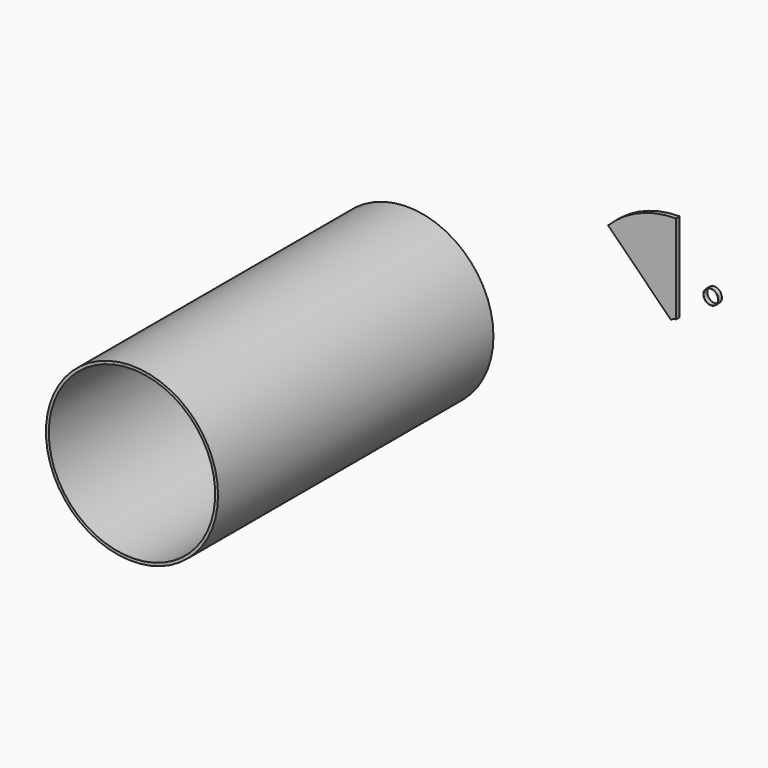
from build123d import *

# Parameters (mm, degrees)
F0_R     = 19.05
F1_DEPTH = 76.2
F3_D     = 36.83
F3_DEPTH = 76.2
F3_TIP   = 11.0648482994
F5_DEPTH = 1.016
F8_R     = 1.651
F8_R_2   = 1.5875
F9_DEPTH = 1.016


# Not quite as in the source:
# - a feature of the source that left no trace in its solid (it failed there, or was rolled back) is left out
# - a length typed as a fraction of an inch, garbled in the dataset ("3 / 203.2 mm" for 3/8 in), is restored
# - a feature names something its author has since deleted; it is built from what else it names


with BuildPart() as f1:
    # F0 (on Front) → F1 (new body)
    with BuildSketch(Plane.XZ):
        with Locations((-13.1577122957, 38.5967120528)):
            Circle(F0_R)
    extrude(amount=F1_DEPTH)

    # F3
    with Locations(Plane.XZ.offset(76.2)):
        with Locations((-13.1577122957, 38.5967120528)):
            Hole(F3_D / 2, depth=F3_DEPTH)
            with Locations((0, 0, -(F3_DEPTH + F3_TIP / 2))):  # 118° drill point
                Cone(0, F3_D / 2, F3_TIP, mode=Mode.SUBTRACT)


with BuildPart() as f5:
    # F4 (on Front) → F5 (new body)
    with BuildSketch(Plane.XZ):
        with BuildLine():
            Line((47.1229890541, 55.69569515), (47.1229890541, 75.38069515))
            ThreePointArc((47.1229890541, 75.38069515), (38.9823557391, 73.7614225053), (32.0810600513, 69.1501241528))
            Line((32.0810600513, 69.1501241528), (46.0004570389, 55.2307271651))
            ThreePointArc((46.0004570389, 55.2307271651), (46.5154791052, 55.5748539078), (47.1229890541, 55.69569515))
        make_face()
    extrude(amount=F5_DEPTH)


with BuildPart() as f9:
    # F8 (on Front) → F9 (new body)
    with BuildSketch(Plane.XZ):
        with Locations((54.8101738095, 62.5820532441)):
            Circle(F8_R)
        with Locations((54.8101738095, 62.5820532441)):
            Circle(F8_R_2, mode=Mode.SUBTRACT)
    extrude(amount=F9_DEPTH)


solid = Compound([f1.part, f5.part, f9.part])
